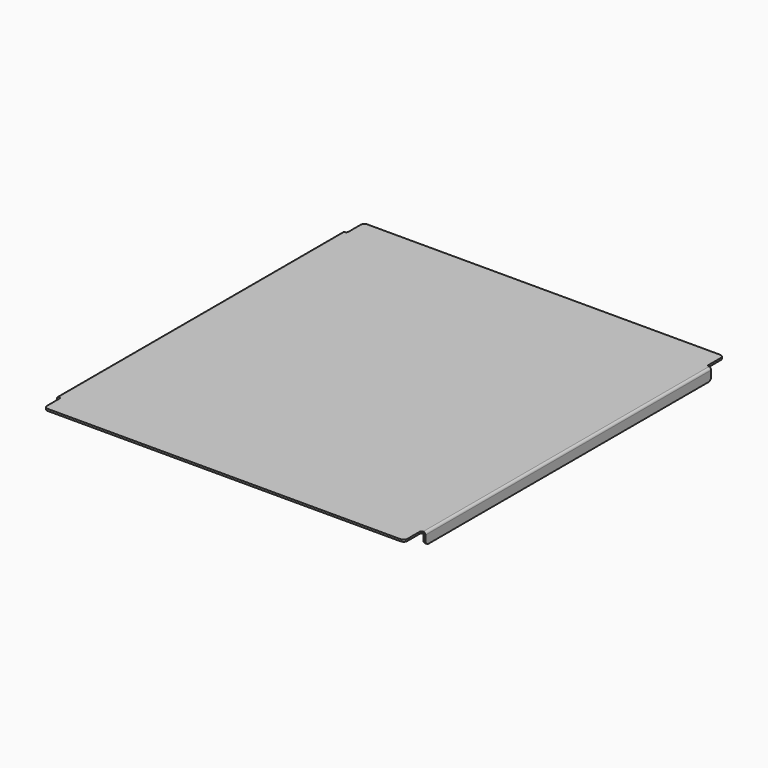
from build123d import *

# Parameters (mm, degrees)
F0_W     = 938
F0_H     = 1040
F1_DEPTH = 5
F3_DEPTH = 465
F4_R     = 10
F5_R     = 5


# Not quite as in the source:
# - a pattern or mirror of a feature is missing from the dataset's text; its kind, count and spacing are read off the source's solid


with BuildPart() as f1:
    # F0 (on Top) → F1 (new body)
    with BuildSketch(Plane.XY):
        Rectangle(F0_W, F0_H)
    extrude(amount=F1_DEPTH)

    # F2 (on Front) → F3 (join, symmetric)
    with BuildSketch(Plane.XZ):
        with BuildLine():
            Line((-469, 0), (-469, 5))
            Line((-469, 5), (-474, 5))
            ThreePointArc((-474, 5), (-478.2426406871, 3.2426406871), (-480, -1))
            Line((-480, -1), (-480, -25))
            Line((-480, -25), (-475, -25))
            Line((-475, -25), (-475, -1))
            ThreePointArc((-475, -1), (-474.7071067812, -0.2928932188), (-474, 0))
            Line((-474, 0), (-469, 0))
        make_face()
    f3 = extrude(amount=F3_DEPTH, both=True)

    # F3_copies: F3 across plane
    add(f3.mirror(Plane(origin=(0, 0, 0), x_dir=(0, 0, 1), z_dir=(1, 0, 0))))

    # F4
    f4_edges = [f1.edges().sort_by_distance(p)[0] for p in [
        (-469, -520, 2.5),
        (-477.5, -465, -25),
        (-477.5, 465, -25),
        (-469, 520, 2.5),
        (469, 520, 2.5),
        (469, -520, 2.5),
        (477.5, -465, -25),
        (477.5, 465, -25),
    ]]
    fillet(f4_edges, radius=F4_R)

    # F5
    f5_edges = [f1.edges().sort_by_distance(p)[0] for p in [
        (-469, -465, 2.5),
        (-469, 465, 2.5),
        (469, -465, 2.5),
        (469, 465, 2.5),
    ]]
    fillet(f5_edges, radius=F5_R)


solid = f1.part
